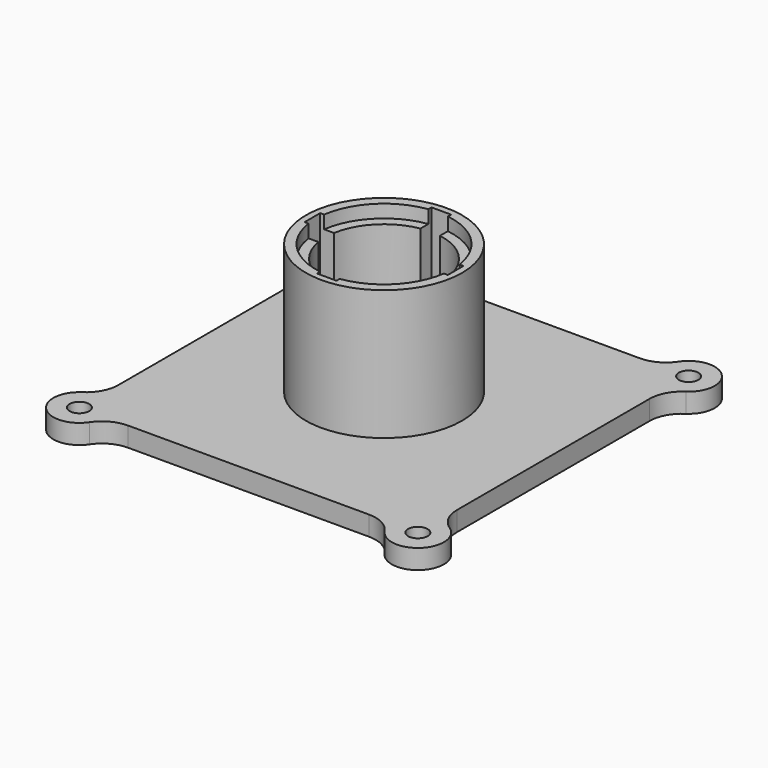
from build123d import *

# Parameters (mm, degrees)
F1_DEPTH = 3
F3_D     = 3
F4_D     = 18
F2_R     = 10.5
F2_R_2   = 9
F5_DEPTH = 18
F2_R_3   = 12
F6_DEPTH = 20
F8_DEPTH = 23.001


with BuildPart() as f1:
    # F0 (on Top) → F1 (new body)
    with BuildSketch(Plane.XY):
        with BuildLine():
            ThreePointArc((-28.2222222222, 22.6740823229), (-26.5904144816, 20.8737078304), (-26, 18.5166852265))
            Line((-26, 18.5166852265), (-26, -18.5166852265))
            ThreePointArc((-26, -18.5166852265), (-26.5904144816, -20.8737078304), (-28.2222222222, -22.6740823229))
            ThreePointArc((-28.2222222222, -22.6740823229), (-28.8284271247, -28.8284271247), (-22.6740823229, -28.2222222222))
            ThreePointArc((-22.6740823229, -28.2222222222), (-20.8737078304, -26.5904144816), (-18.5166852265, -26))
            Line((-18.5166852265, -26), (18.5166852265, -26))
            ThreePointArc((18.5166852265, -26), (20.8737078304, -26.5904144816), (22.6740823229, -28.2222222222))
            ThreePointArc((22.6740823229, -28.2222222222), (28.8284271247, -28.8284271247), (28.2222222222, -22.6740823229))
            ThreePointArc((28.2222222222, -22.6740823229), (26.5904144816, -20.8737078304), (26, -18.5166852265))
            Line((26, -18.5166852265), (26, 18.5166852265))
            ThreePointArc((26, 18.5166852265), (26.5904144816, 20.8737078304), (28.2222222222, 22.6740823229))
            ThreePointArc((28.2222222222, 22.6740823229), (28.8284271247, 28.8284271247), (22.6740823229, 28.2222222222))
            ThreePointArc((22.6740823229, 28.2222222222), (20.8737078304, 26.5904144816), (18.5166852265, 26))
            Line((18.5166852265, 26), (-18.5166852265, 26))
            ThreePointArc((-18.5166852265, 26), (-20.8737078304, 26.5904144816), (-22.6740823229, 28.2222222222))
            ThreePointArc((-22.6740823229, 28.2222222222), (-28.8284271247, 28.8284271247), (-28.2222222222, 22.6740823229))
        make_face()
    extrude(amount=F1_DEPTH)

    # F3 (through all)
    with Locations(Plane.XY.offset(3)):
        with Locations((26, 26), (-26, 26), (-26, -26), (26, -26)):
            Hole(F3_D / 2)

    # F4 (through all)
    with Locations(Plane.XY.offset(3)):
        with Locations((0, 0)):
            Hole(F4_D / 2)

    # F2 (on face) → F5 (join)
    with BuildSketch(Plane.XY.offset(3)):
        Circle(F2_R)
        Circle(F2_R_2, mode=Mode.SUBTRACT)
    extrude(amount=F5_DEPTH)

    # F2 (on face) → F6 (join)
    with BuildSketch(Plane.XY.offset(3)):
        Circle(F2_R_3)
        Circle(F2_R, mode=Mode.SUBTRACT)
    extrude(amount=F6_DEPTH)

    # F7 (on face) → F8 (cut, through all)
    with BuildSketch(Plane.XY.offset(23)):
        with BuildLine():
            Line((-10.3923048454, 1.5), (-11, 1.5))
            Line((-11, 1.5), (-11, -1.5))
            Line((-11, -1.5), (-10.3923048454, -1.5))
            ThreePointArc((-10.3923048454, -1.5), (-10.5, 0), (-10.3923048454, 1.5))
        make_face()
        with BuildLine():
            Line((-1.5, 1.5), (-10.3923048454, 1.5))
            ThreePointArc((-10.3923048454, 1.5), (-10.5, 0), (-10.3923048454, -1.5))
            Line((-10.3923048454, -1.5), (-1.5, -1.5))
            Line((-1.5, -1.5), (-1.5, 1.5))
        make_face()
        with BuildLine():
            Line((1.5, -1.5), (-1.5, -1.5))
            Line((-1.5, -1.5), (-1.5, -10.3923048454))
            ThreePointArc((-1.5, -10.3923048454), (0, -10.5), (1.5, -10.3923048454))
            Line((1.5, -10.3923048454), (1.5, -1.5))
        make_face()
        with BuildLine():
            ThreePointArc((1.5, -10.3923048454), (0, -10.5), (-1.5, -10.3923048454))
            Line((-1.5, -10.3923048454), (-1.5, -11))
            Line((-1.5, -11), (1.5, -11))
            Line((1.5, -11), (1.5, -10.3923048454))
        make_face()
        with BuildLine():
            Line((10.3923048454, 1.5), (1.5, 1.5))
            Line((1.5, 1.5), (1.5, -1.5))
            Line((1.5, -1.5), (10.3923048454, -1.5))
            ThreePointArc((10.3923048454, -1.5), (10.473041604, -0.7519305564), (10.5, 0))
            ThreePointArc((10.5, 0), (10.473041604, 0.7519305564), (10.3923048454, 1.5))
        make_face()
        with BuildLine():
            Line((11, 1.5), (10.3923048454, 1.5))
            ThreePointArc((10.3923048454, 1.5), (10.473041604, 0.7519305564), (10.5, 0))
            ThreePointArc((10.5, 0), (10.473041604, -0.7519305564), (10.3923048454, -1.5))
            Line((10.3923048454, -1.5), (11, -1.5))
            Line((11, -1.5), (11, 1.5))
        make_face()
        with BuildLine():
            Line((-1.5, 10.3923048454), (-1.5, 1.5))
            Line((-1.5, 1.5), (1.5, 1.5))
            Line((1.5, 1.5), (1.5, 10.3923048454))
            ThreePointArc((1.5, 10.3923048454), (0, 10.5), (-1.5, 10.3923048454))
        make_face()
        with BuildLine():
            Line((-1.5, 11), (-1.5, 10.3923048454))
            ThreePointArc((-1.5, 10.3923048454), (0, 10.5), (1.5, 10.3923048454))
            Line((1.5, 10.3923048454), (1.5, 11))
            Line((1.5, 11), (-1.5, 11))
        make_face()
    extrude(amount=-F8_DEPTH, mode=Mode.SUBTRACT)


with BuildPart() as f9_1:
    # F9: copy of F1
    add(f1.part)


solid = Compound([f1.part, f9_1.part])
